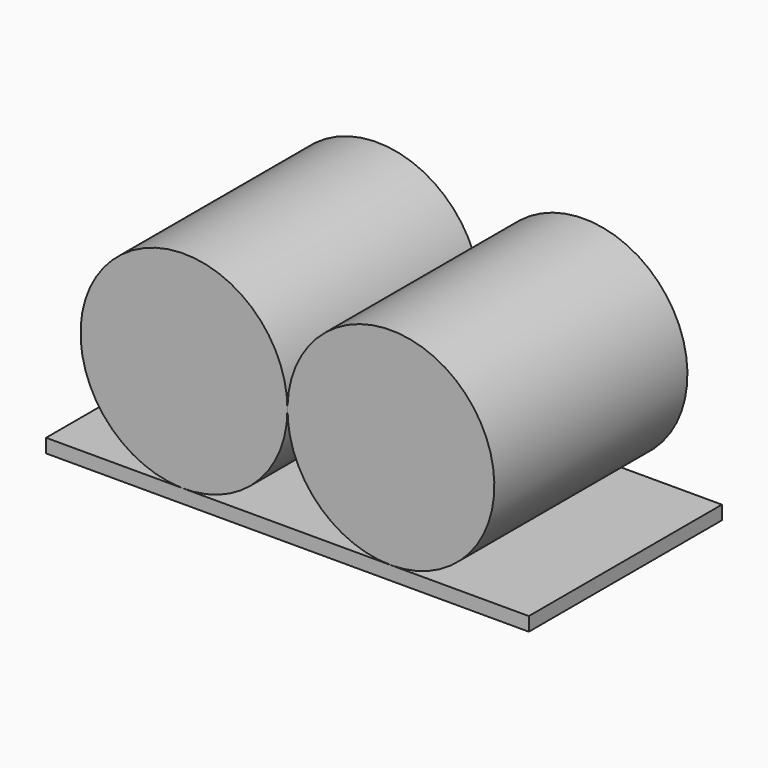
from build123d import *

# Parameters (mm, degrees)
F1_DEPTH = 88.9


# Not quite as in the source:
# - a feature names something its author has since deleted; it is built from what else it names


with BuildPart() as f1:
    # F0 (on Front) → F1 (new body)
    with BuildSketch(Plane.XZ):
        with BuildLine():
            ThreePointArc((-38.1, -45.8680424225), (-11.1592316368, -34.7088107857), (0, -7.7680424225))
            ThreePointArc((0, -7.7680424225), (-65.0407683632, 19.1727259407), (-38.1, -45.8680424225))
        make_face()
    extrude(amount=F1_DEPTH)


with BuildPart() as f1b:
    # F0 (on Front) → F1, piece 2 (new body)
    with BuildSketch(Plane.XZ):
        with BuildLine():
            ThreePointArc((76.2, -7.7680424225), (38.1, 30.3319575775), (0, -7.7680424225))
            ThreePointArc((0, -7.7680424225), (11.1592316368, -34.7088107857), (38.1, -45.8680424225))
            ThreePointArc((38.1, -45.8680424225), (65.0407683632, -34.7088107857), (76.2, -7.7680424225))
        make_face()
    extrude(amount=F1_DEPTH)


with BuildPart() as f1c:
    # F0 (on Front) → F1, piece 3 (new body)
    with BuildSketch(Plane.XZ):
        Polygon((38.1, -45.8680424225), (-38.1, -45.8680424225), (-88.9, -45.8680424225), (-88.9, -50.9480424225), (88.9, -50.9480424225), (88.9, -45.8680424225), align=None)
    extrude(amount=F1_DEPTH)


solid = Compound([f1.part, f1b.part, f1c.part])
